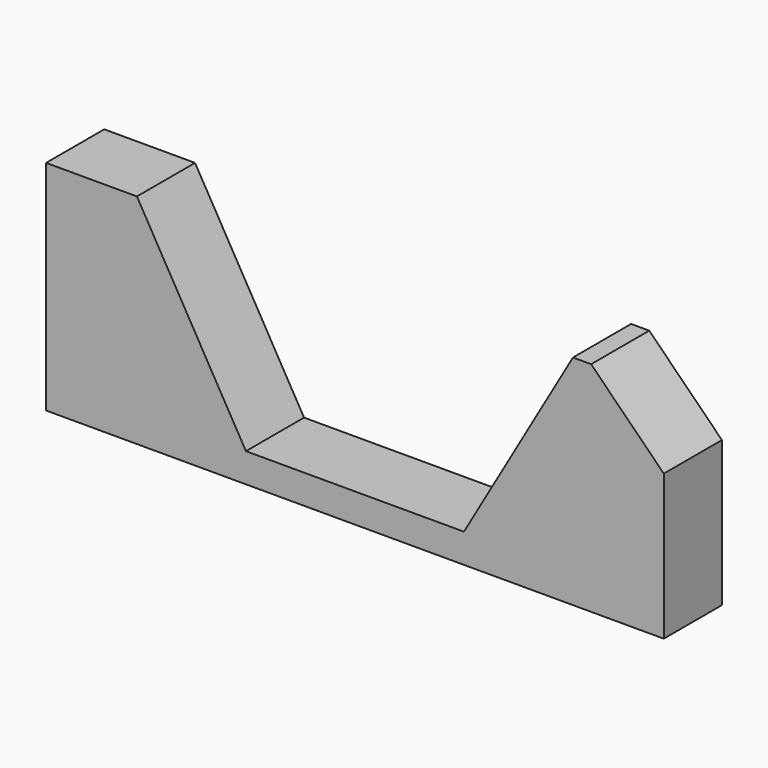
from build123d import *

# Parameters (mm, degrees)
F1_DEPTH    = 116.84
F2_W        = 86.36
F2_H        = 15.24
F3_DEPTH    = 2.54
F4_W        = 86.36
F4_H        = 15.24
F5_DEPTH    = 2.54
F6_T1_DEPTH = 148.0482991577
F6_T3_DEPTH = 112.4882991577
F7_SIZE     = 5.08
F8_W        = 91.7793288827
F8_H        = 30.2478149533
F9_DEPTH    = 106.68
F10_W       = 99.2863364518
F10_H       = 25.3497036174
F11_DEPTH   = 10.16
F12_W       = 15.3326203581
F12_H       = 21.305212751
F13_DEPTH   = 43.18


# Not quite as in the source:
# - a fillet or chamfer that OpenCascade refuses, or shapes differently, is made with other operations: its cross-section is extruded or revolved along the edge and cut away or added


with BuildPart() as f1:
    # F0 (on Front) → F1 (new body)
    with BuildSketch(Plane.XZ):
        Polygon((43.18, 0), (36.83, 0), (29.21, -13.1982271537), (13.97, -13.1982271537), (6.35, 0), (0, 0), (-6.35, 0), (-13.97, -13.1982271537), (-29.21, -13.1982271537), (-36.83, 0), (-43.18, 0), (-43.18, -15.24), (0, -15.24), (43.18, -15.24), align=None)
    extrude(amount=F1_DEPTH)

    # F2 (on face) → F3 (join)
    with BuildSketch(Plane.XZ.offset(116.84)):
        with Locations((0, -7.62)):
            Rectangle(F2_W, F2_H)
    extrude(amount=F3_DEPTH)

    # F4 (on face) → F5 (join)
    with BuildSketch(Plane(origin=(0, 0, 0), x_dir=(-1, 0, 0), z_dir=(0, 1, 0))):
        with Locations((0, -7.62)):
            Rectangle(F4_W, F4_H)
    extrude(amount=F5_DEPTH)

    # F6: chamfer of 5.08 on 4 edges, made by hand

    # F6_s2 → F6_t1 (cut)
    with BuildSketch(Plane.XZ.offset(-15.6041495789)):
        Polygon((-38.1, 0), (-43.18, -5.08), (-43.18, 0), align=None)
        Polygon((38.1, 0), (43.18, -5.08), (43.18, 0), align=None)
    extrude(amount=F6_T1_DEPTH, mode=Mode.SUBTRACT)

    # F6_s4 → F6_t3 (cut)
    with BuildSketch(Plane.YZ.offset(-56.2441495789)):
        Polygon((-114.3, 0), (-119.38, -5.08), (-119.38, 0), align=None)
        Polygon((-2.54, 0), (2.54, -5.08), (2.54, 0), align=None)
    extrude(amount=F6_T3_DEPTH, mode=Mode.SUBTRACT)

    # F7
    f7_edges = [f1.edges().sort_by_distance(p)[0] for p in [
        (-43.18, -119.38, -10.16),
        (43.18, -119.38, -10.16),
        (43.18, 2.54, -10.16),
        (-43.18, 2.54, -10.16),
    ]]
    chamfer(f7_edges, length=F7_SIZE)

    # F8 (on face) → F9 (cut)
    with BuildSketch(Plane.XZ.offset(119.38)):
        with Locations((-0.610165298, -4.9024894834)):
            Rectangle(F8_W, F8_H)
    extrude(amount=-F9_DEPTH, mode=Mode.SUBTRACT)

    # F10 (on face) → F11 (cut)
    with BuildSketch(Plane(origin=(0, 2.54, 0), x_dir=(-1, 0, 0), z_dir=(0, 1, 0))):
        with Locations((1.3202968985, -7.6577230357)):
            Rectangle(F10_W, F10_H)
    extrude(amount=-F11_DEPTH, mode=Mode.SUBTRACT)

    # F12 (on face) → F13 (cut)
    with BuildSketch(Plane(origin=(-43.18, 0, 0), x_dir=(0, -1, 0), z_dir=(-1, 0, 0))):
        with Locations((10.5058533372, -7.6547963545)):
            Rectangle(F12_W, F12_H)
    extrude(amount=-F13_DEPTH, mode=Mode.SUBTRACT)


solid = f1.part
